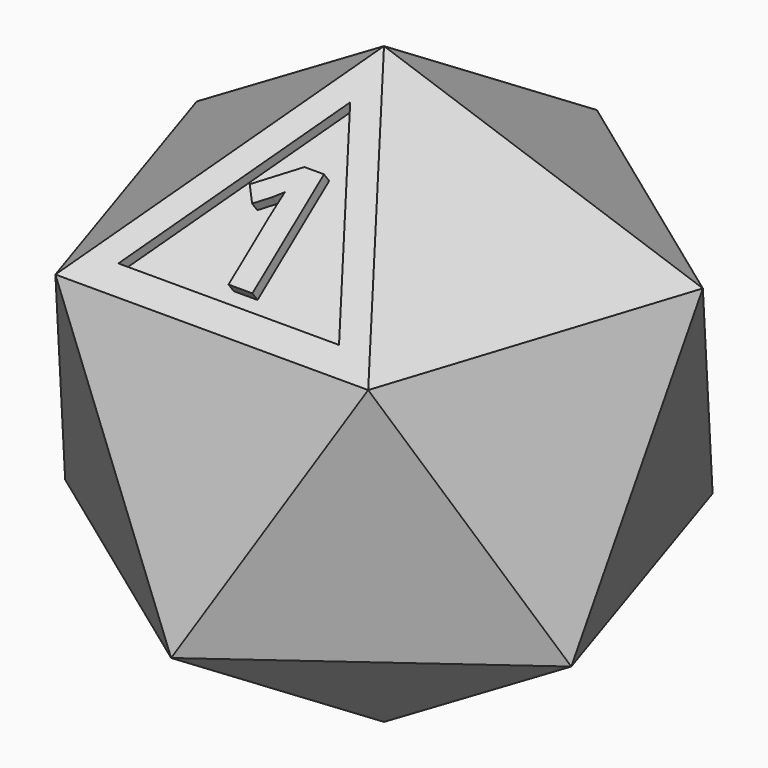
from build123d import *

# Parameters (mm, degrees)
F12_DEPTH      = 37.3243635206
F12_DEPTH_BACK = 37.3243635206
F15_DEPTH      = 37.3243635206
F15_DEPTH_BACK = 37.3243635206
F18_DEPTH      = 37.3243635206
F18_DEPTH_BACK = 37.3243635206
F21_DEPTH      = 37.3243635206
F21_DEPTH_BACK = 37.3243635206
F24_DEPTH      = 37.3243635206
F24_DEPTH_BACK = 37.3243635206
F28_DEPTH      = 99.1671965959
F28_DEPTH_BACK = 99.1671965959
F32_DEPTH      = 89.4601183415
F32_DEPTH_BACK = 89.4601183415
F35_DEPTH      = 89.4601183415
F35_DEPTH_BACK = 88.5596960493
F39_DEPTH      = 99.1671965959
F39_DEPTH_BACK = 96.8098604305
F42_DEPTH      = 68.0823305395
F42_DEPTH_BACK = 70.9961582856
F45_DEPTH      = 92.4043169267
F45_DEPTH_BACK = 99.1671965959
F48_DEPTH      = 81.4313769211
F48_DEPTH_BACK = 89.4601183415
F52_DEPTH      = 88.5596960493
F52_DEPTH_BACK = 82.3317992133
F56_DEPTH      = 92.4043169267
F56_DEPTH_BACK = 96.8098604305
F59_DEPTH      = 68.0823305395
F59_DEPTH_BACK = 68.0823305395
F62_DEPTH      = 37.3243635206
F62_DEPTH_BACK = 37.3243635206
F65_DEPTH      = 68.0823305395
F65_DEPTH_BACK = 68.0823305395
F68_DEPTH      = 81.4313769211
F68_DEPTH_BACK = 81.4313769211
F71_DEPTH      = 92.4043169267
F71_DEPTH_BACK = 92.4043169267
F74_DEPTH      = 92.4043169267
F74_DEPTH_BACK = 92.4043169267
F76_DEPTH      = 2.54
F78_DEPTH      = 2.54


# Not quite as in the source:
# - a feature names something its author has since deleted; it is built from what else it names


with BuildPart() as f9:
    # F7 (on Front) → F9 (revolve)
    with BuildSketch(Plane.XZ):
        with BuildLine():
            Line((0, 0), (0, 31.75))
            Line((0, 31.75), (0, 70.9951582856))
            ThreePointArc((0, 70.9951582856), (-70.9951582856, 0), (0, -70.9951582856))
            Line((0, -70.9951582856), (0, -31.75))
            Line((0, -31.75), (0, 0))
        make_face()
    revolve(axis=Axis((0, 0, -35.4975791428), (0, 0, -1)))

    # F11 (on 3pt) → F12 (cut, two sides)
    with BuildSketch(Plane(origin=(0, 0, 0), x_dir=(-0.5877852523, 0.8090169944, 0), z_dir=(0.8090169944, 0.5877852523, 0))) as f12_sk:
        Polygon((-63.5, -70.9951582856), (0, -70.9951582856), (-51.3725791428, -31.75), (-63.5, -31.75), align=None)
    extrude(amount=F12_DEPTH, mode=Mode.SUBTRACT)
    extrude(f12_sk.sketch, amount=-F12_DEPTH_BACK, mode=Mode.SUBTRACT)

    # F14 (on 3pt) → F15 (cut, two sides)
    with BuildSketch(Plane(origin=(0, 0, 0), x_dir=(-0.5877852523, -0.8090169944, 0), z_dir=(-0.8090169944, 0.5877852523, 0))) as f15_sk:
        Polygon((51.3725791428, -31.75), (0, -70.9951582856), (63.5, -70.9951582856), (63.5, -31.75), align=None)
    extrude(amount=-F15_DEPTH, mode=Mode.SUBTRACT)
    extrude(f15_sk.sketch, amount=F15_DEPTH_BACK, mode=Mode.SUBTRACT)

    # F17 (on 3pt) → F18 (cut, two sides)
    with BuildSketch(Plane(origin=(0, 0, 0), x_dir=(0.9510565163, -0.3090169944, 0), z_dir=(-0.3090169944, -0.9510565163, 0))) as f18_sk:
        Polygon((-63.5, -70.9951582856), (0, -70.9951582856), (-51.3725791428, -31.75), (-63.5, -31.75), align=None)
    extrude(amount=-F18_DEPTH, mode=Mode.SUBTRACT)
    extrude(f18_sk.sketch, amount=F18_DEPTH_BACK, mode=Mode.SUBTRACT)

    # F20 (on 3pt) → F21 (cut, two sides)
    with BuildSketch(Plane.YZ) as f21_sk:
        Polygon((51.3725791428, -31.75), (0, -70.9951582856), (63.5, -70.9951582856), (63.5, -31.75), align=None)
    extrude(amount=-F21_DEPTH, mode=Mode.SUBTRACT)
    extrude(f21_sk.sketch, amount=F21_DEPTH_BACK, mode=Mode.SUBTRACT)

    # F23 (on 3pt) → F24 (cut, two sides)
    with BuildSketch(Plane(origin=(0, 0, 0), x_dir=(-0.9510565163, -0.3090169944, 0), z_dir=(-0.3090169944, 0.9510565163, 0))) as f24_sk:
        Polygon((-63.5, -70.9951582856), (0, -70.9951582856), (-51.3725791428, -31.75), (-63.5, -31.75), align=None)
    extrude(amount=F24_DEPTH, mode=Mode.SUBTRACT)
    extrude(f24_sk.sketch, amount=-F24_DEPTH_BACK, mode=Mode.SUBTRACT)

    # F27 (on 3pt) → F28 (cut, two sides)
    with BuildSketch(Plane(origin=(0, 0, 0), x_dir=(-0.5877852523, 0.8090169944, 0), z_dir=(0.8090169944, 0.5877852523, 0))) as f28_sk:
        Polygon((-70.9951582856, -31.75), (-51.3725791428, -31.75), (-63.5, 31.75), (-70.9951582856, 31.75), align=None)
    extrude(amount=F28_DEPTH, mode=Mode.SUBTRACT)
    extrude(f28_sk.sketch, amount=-F28_DEPTH_BACK, mode=Mode.SUBTRACT)

    # F31 (on 3pt) → F32 (cut, two sides)
    with BuildSketch(Plane(origin=(0, 0, 0), x_dir=(0.9510565163, -0.3090169944, 0), z_dir=(-0.3090169944, -0.9510565163, 0))) as f32_sk:
        Polygon((70.9951582856, 31.75), (51.3725791428, 31.75), (63.5, -31.75), (70.9951582856, -31.75), align=None)
    extrude(amount=-F32_DEPTH, mode=Mode.SUBTRACT)
    extrude(f32_sk.sketch, amount=F32_DEPTH_BACK, mode=Mode.SUBTRACT)

    # F34 (on 3pt) → F35 (cut, two sides)
    with BuildSketch(Plane(origin=(0, 0, 0), x_dir=(0.9510565163, 0.3090169944, 0), z_dir=(0.3090169944, -0.9510565163, 0))) as f35_sk:
        Polygon((63.5, 31.75), (51.3725791428, -31.75), (70.9951582856, -31.75), (70.9951582856, 31.75), align=None)
    extrude(amount=-F35_DEPTH, mode=Mode.SUBTRACT)
    extrude(f35_sk.sketch, amount=F35_DEPTH_BACK, mode=Mode.SUBTRACT)

    # F38 (on 3pt) → F39 (cut, two sides)
    with BuildSketch(Plane(origin=(0, 0, 0), x_dir=(0.5877852523, 0.8090169944, 0), z_dir=(0.8090169944, -0.5877852523, 0))) as f39_sk:
        Polygon((70.9951582856, 31.75), (51.3725791428, 31.75), (63.5, -31.75), (70.9951582856, -31.75), align=None)
    extrude(amount=-F39_DEPTH, mode=Mode.SUBTRACT)
    extrude(f39_sk.sketch, amount=F39_DEPTH_BACK, mode=Mode.SUBTRACT)

    # F41 (on 3pt) → F42 (cut, two sides)
    with BuildSketch(Plane(origin=(0, 0, 0), x_dir=(0, -1, 0), z_dir=(-1, 0, 0))) as f42_sk:
        Polygon((-70.9951582856, -31.75), (-51.3725791428, -31.75), (-63.5, 31.75), (-70.9951582856, 31.75), align=None)
    extrude(amount=-F42_DEPTH, mode=Mode.SUBTRACT)
    extrude(f42_sk.sketch, amount=F42_DEPTH_BACK, mode=Mode.SUBTRACT)

    # F44 (on 3pt) → F45 (cut, two sides)
    with BuildSketch(Plane(origin=(0, 0, 0), x_dir=(0.5877852523, -0.8090169944, 0), z_dir=(-0.8090169944, -0.5877852523, 0))) as f45_sk:
        Polygon((-63.5, -31.75), (-51.3725791428, 31.75), (-70.9951582856, 31.75), (-70.9951582856, -31.75), align=None)
    extrude(amount=-F45_DEPTH, mode=Mode.SUBTRACT)
    extrude(f45_sk.sketch, amount=F45_DEPTH_BACK, mode=Mode.SUBTRACT)

    # F47 (on 3pt) → F48 (cut, two sides)
    with BuildSketch(Plane(origin=(0, 0, 0), x_dir=(0.9510565163, -0.3090169944, 0), z_dir=(-0.3090169944, -0.9510565163, 0))) as f48_sk:
        Polygon((-70.9951582856, -31.75), (-51.3725791428, -31.75), (-63.5, 31.75), (-70.9951582856, 31.75), align=None)
    extrude(amount=-F48_DEPTH, mode=Mode.SUBTRACT)
    extrude(f48_sk.sketch, amount=F48_DEPTH_BACK, mode=Mode.SUBTRACT)

    # F51 (on 3pt) → F52 (cut, two sides)
    with BuildSketch(Plane(origin=(0, 0, 0), x_dir=(-0.9510565163, -0.3090169944, 0), z_dir=(-0.3090169944, 0.9510565163, 0))) as f52_sk:
        Polygon((70.9951582856, 31.75), (51.3725791428, 31.75), (63.5, -31.75), (70.9951582856, -31.75), align=None)
    extrude(amount=-F52_DEPTH, mode=Mode.SUBTRACT)
    extrude(f52_sk.sketch, amount=F52_DEPTH_BACK, mode=Mode.SUBTRACT)

    # F55 (on 3pt) → F56 (cut, two sides)
    with BuildSketch(Plane(origin=(0, 0, 0), x_dir=(0.5877852523, 0.8090169944, 0), z_dir=(0.8090169944, -0.5877852523, 0))) as f56_sk:
        Polygon((-70.9951582856, -31.75), (-51.3725791428, -31.75), (-63.5, 31.75), (-70.9951582856, 31.75), align=None)
    extrude(amount=-F56_DEPTH, mode=Mode.SUBTRACT)
    extrude(f56_sk.sketch, amount=F56_DEPTH_BACK, mode=Mode.SUBTRACT)

    # F58 (on 3pt) → F59 (cut, two sides)
    with BuildSketch(Plane(origin=(0, 0, 0), x_dir=(0, -1, 0), z_dir=(-1, 0, 0))) as f59_sk:
        Polygon((70.9951582856, 31.75), (51.3725791428, 31.75), (63.5, -31.75), (70.9951582856, -31.75), align=None)
    extrude(amount=-F59_DEPTH, mode=Mode.SUBTRACT)
    extrude(f59_sk.sketch, amount=F59_DEPTH_BACK, mode=Mode.SUBTRACT)

    # F61 (on 3pt) → F62 (cut, two sides)
    with BuildSketch(Plane(origin=(0, 0, 0), x_dir=(0.9510565163, -0.3090169944, 0), z_dir=(-0.3090169944, -0.9510565163, 0))) as f62_sk:
        Polygon((63.5, 70.9951582856), (0, 70.9951582856), (51.3725791428, 31.75), (63.5, 31.75), align=None)
    extrude(amount=F62_DEPTH, mode=Mode.SUBTRACT)
    extrude(f62_sk.sketch, amount=-F62_DEPTH_BACK, mode=Mode.SUBTRACT)

    # F64 (on 3pt) → F65 (cut, two sides)
    with BuildSketch(Plane.YZ) as f65_sk:
        Polygon((-51.3725791428, 31.75), (0, 70.9951582856), (-63.5, 70.9951582856), (-63.5, 31.75), align=None)
    extrude(amount=-F65_DEPTH, mode=Mode.SUBTRACT)
    extrude(f65_sk.sketch, amount=F65_DEPTH_BACK, mode=Mode.SUBTRACT)

    # F67 (on 3pt) → F68 (cut, two sides)
    with BuildSketch(Plane(origin=(0, 0, 0), x_dir=(0.9510565163, 0.3090169944, 0), z_dir=(0.3090169944, -0.9510565163, 0))) as f68_sk:
        Polygon((-51.3725791428, 31.75), (0, 70.9951582856), (-63.5, 70.9951582856), (-63.5, 31.75), align=None)
    extrude(amount=-F68_DEPTH, mode=Mode.SUBTRACT)
    extrude(f68_sk.sketch, amount=F68_DEPTH_BACK, mode=Mode.SUBTRACT)

    # F70 (on 3pt) → F71 (cut, two sides)
    with BuildSketch(Plane(origin=(0, 0, 0), x_dir=(-0.5877852523, 0.8090169944, 0), z_dir=(0.8090169944, 0.5877852523, 0))) as f71_sk:
        Polygon((63.5, 70.9951582856), (0, 70.9951582856), (51.3725791428, 31.75), (63.5, 31.75), align=None)
    extrude(amount=-F71_DEPTH, mode=Mode.SUBTRACT)
    extrude(f71_sk.sketch, amount=F71_DEPTH_BACK, mode=Mode.SUBTRACT)

    # F73 (on 3pt) → F74 (cut, two sides)
    with BuildSketch(Plane(origin=(0, 0, 0), x_dir=(0.5877852523, 0.8090169944, 0), z_dir=(0.8090169944, -0.5877852523, 0))) as f74_sk:
        Polygon((63.5, 70.9951582856), (0, 70.9951582856), (51.3725791428, 31.75), (63.5, 31.75), align=None)
    extrude(amount=-F74_DEPTH, mode=Mode.SUBTRACT)
    extrude(f74_sk.sketch, amount=F74_DEPTH_BACK, mode=Mode.SUBTRACT)

    # F75 (on face) → F76 (cut)
    with BuildSketch(Plane(origin=(0, -34.2483860952, 44.8317194285), x_dir=(1, 0, 0), z_dir=(0, -0.6070619982, 0.7946544723))):
        Polygon((26.3258408925, -15.1992313259), (0, 30.3984626519), (-26.3258408925, -15.1992313259), align=None)
        with BuildLine():
            Line((3.3501555036, 15.3069211224), (3.3501555036, -11.5860768557))
            Line((3.3501555036, -11.5860768557), (-2.335691738, -11.5860768557))
            Line((-2.335691738, -11.5860768557), (-2.335691738, 3.9764284308))
            Line((-2.335691738, 3.9764284308), (-2.2768320357, 6.5309395104))
            Line((-2.2768320357, 6.5309395104), (-2.1885424823, 9.3267753694))
            add(Edge.make_bspline(
                [(-2.1885424823, 9.3267753694), (-3.6011753374, 7.9141425143), (-4.1544565389, 7.4726947471)],
                knots=[0, 0, 0, 1, 1, 1], degree=2))
            Line((-4.1544565389, 7.4726947471), (-7.2445909094, 4.9888153103))
            Line((-7.2445909094, 4.9888153103), (-9.9874530363, 8.4085640136))
            Line((-9.9874530363, 8.4085640136), (-1.3233048586, 15.3069211224))
            Line((-1.3233048586, 15.3069211224), (3.3501555036, 15.3069211224))
        make_face(mode=Mode.SUBTRACT)
    extrude(amount=-F76_DEPTH, mode=Mode.SUBTRACT)

    # F77 (on face) → F78 (cut)
    with BuildSketch(Plane(origin=(0, 34.2483860952, -44.8317194285), x_dir=(1, 0, 0), z_dir=(0, 0.6070619982, -0.7946544723))):
        with BuildLine():
            Line((26.3258408925, -15.1992313259), (0, 30.3984626519))
            Line((0, 30.3984626519), (-11.6958512292, 10.1406540851))
            add(Edge.make_bspline(
                [(-11.6958512292, 10.1406540851), (-10.9085633152, 10.5210577591), (-10.0027118644, 10.7419129699)],
                knots=[0.151662927, 0.151662927, 0.151662927, 1, 1, 1], degree=2))
            add(Edge.make_bspline(
                [(-10.0027118644, 10.7419129699), (-8.9349152542, 11.002251953), (-7.6128813559, 11.002251953)],
                knots=[0, 0, 0, 1, 1, 1], degree=2))
            add(Edge.make_bspline(
                [(-7.6128813559, 11.002251953), (-5.8718644068, 11.002251953), (-4.5376271186, 10.3676756818)],
                knots=[0, 0, 0, 1, 1, 1], degree=2))
            add(Edge.make_bspline(
                [(-4.5376271186, 10.3676756818), (-3.2033898305, 9.7330994106), (-2.4650847458, 8.5880146649)],
                knots=[0, 0, 0, 1, 1, 1], degree=2))
            add(Edge.make_bspline(
                [(-2.4650847458, 8.5880146649), (-1.726779661, 7.4429299191), (-1.726779661, 5.9703875462)],
                knots=[0, 0, 0, 1, 1, 1], degree=2))
            add(Edge.make_bspline(
                [(-1.726779661, 5.9703875462), (-1.726779661, 4.6849638174), (-2.1783050847, 3.5602180547)],
                knots=[0, 0, 0, 1, 1, 1], degree=2))
            add(Edge.make_bspline(
                [(-2.1783050847, 3.5602180547), (-2.6298305085, 2.435472292), (-3.5776271186, 1.2537773767)],
                knots=[0, 0, 0, 1, 1, 1], degree=2))
            add(Edge.make_bspline(
                [(-3.5776271186, 1.2537773767), (-4.5254237288, 0.0720824615), (-6.913220339, -2.1163921148)],
                knots=[0, 0, 0, 1, 1, 1], degree=2))
            Line((-6.913220339, -2.1163921148), (-9.3050847458, -4.3658836402))
            Line((-9.3050847458, -4.3658836402), (-9.3050847458, -4.5407988945))
            Line((-9.3050847458, -4.5407988945), (-1.2061016949, -4.5407988945))
            Line((-1.2061016949, -4.5407988945), (-1.2061016949, -7.8479175385))
            Line((-1.2061016949, -7.8479175385), (-14.1986440678, -7.8479175385))
            Line((-14.1986440678, -7.8479175385), (-14.1986440678, -5.1143582165))
            Line((-14.1986440678, -5.1143582165), (-9.5328813559, -0.3997819453))
            add(Edge.make_bspline(
                [(-9.5328813559, -0.3997819453), (-7.4583050847, 1.7236078852), (-6.8237288136, 2.5432689022)],
                knots=[0, 0, 0, 1, 1, 1], degree=2))
            add(Edge.make_bspline(
                [(-6.8237288136, 2.5432689022), (-6.1891525424, 3.3629299191), (-5.9084745763, 4.0625909361)],
                knots=[0, 0, 0, 1, 1, 1], degree=2))
            add(Edge.make_bspline(
                [(-5.9084745763, 4.0625909361), (-5.6277966102, 4.762251953), (-5.6277966102, 5.5107265293)],
                knots=[0, 0, 0, 1, 1, 1], degree=2))
            add(Edge.make_bspline(
                [(-5.6277966102, 5.5107265293), (-5.6277966102, 6.6293705971), (-6.2461016949, 7.1764892411)],
                knots=[0, 0, 0, 1, 1, 1], degree=2))
            add(Edge.make_bspline(
                [(-6.2461016949, 7.1764892411), (-6.8644067797, 7.7236078852), (-7.893559322, 7.7236078852)],
                knots=[0, 0, 0, 1, 1, 1], degree=2))
            add(Edge.make_bspline(
                [(-7.893559322, 7.7236078852), (-8.9715254237, 7.7236078852), (-9.9884745763, 7.2273366988)],
                knots=[0, 0, 0, 1, 1, 1], degree=2))
            add(Edge.make_bspline(
                [(-9.9884745763, 7.2273366988), (-11.0054237288, 6.7310655123), (-12.1118644068, 5.815811275)],
                knots=[0, 0, 0, 1, 1, 1], degree=2))
            Line((-12.1118644068, 5.815811275), (-13.3475580235, 7.2798139981))
            Line((-13.3475580235, 7.2798139981), (-26.3258408925, -15.1992313259))
            Line((-26.3258408925, -15.1992313259), (26.3258408925, -15.1992313259))
        make_face()
        with BuildLine():
            add(Edge.make_bspline(
                [(11.906440678, 8.5900485632), (13.5518644068, 6.1493705971), (13.5518644068, 1.4429299191)],
                knots=[0, 0, 0, 1, 1, 1], degree=2))
            add(Edge.make_bspline(
                [(13.5518644068, 1.4429299191), (13.5518644068, -3.4221548267), (11.9572881356, -5.7631717758)],
                knots=[0, 0, 0, 1, 1, 1], degree=2))
            add(Edge.make_bspline(
                [(11.9572881356, -5.7631717758), (10.3627118644, -8.104188725), (7.0433898305, -8.104188725)],
                knots=[0, 0, 0, 1, 1, 1], degree=2))
            add(Edge.make_bspline(
                [(7.0433898305, -8.104188725), (3.8257627119, -8.104188725), (2.1925423729, -5.6879175385)],
                knots=[0, 0, 0, 1, 1, 1], degree=2))
            add(Edge.make_bspline(
                [(2.1925423729, -5.6879175385), (0.5593220339, -3.2716463521), (0.5593220339, 1.4429299191)],
                knots=[0, 0, 0, 1, 1, 1], degree=2))
            add(Edge.make_bspline(
                [(0.5593220339, 1.4429299191), (0.5593220339, 6.3649638174), (2.1498305085, 8.6978451733)],
                knots=[0, 0, 0, 1, 1, 1], degree=2))
            add(Edge.make_bspline(
                [(2.1498305085, 8.6978451733), (3.7403389831, 11.0307265293), (7.0433898305, 11.0307265293)],
                knots=[0, 0, 0, 1, 1, 1], degree=2))
            add(Edge.make_bspline(
                [(7.0433898305, 11.0307265293), (10.2610169492, 11.0307265293), (11.906440678, 8.5900485632)],
                knots=[0, 0, 0, 1, 1, 1], degree=2))
        make_face(mode=Mode.SUBTRACT)
        with BuildLine():
            add(Edge.make_bspline(
                [(5.0603389831, 6.3568282242), (4.4644067797, 4.8639468683), (4.4644067797, 1.4429299191)],
                knots=[0, 0, 0, 1, 1, 1], degree=2))
            add(Edge.make_bspline(
                [(4.4644067797, 1.4429299191), (4.4644067797, -1.9740192334), (5.0542372881, -3.4546971995)],
                knots=[0, 0, 0, 1, 1, 1], degree=2))
            add(Edge.make_bspline(
                [(5.0542372881, -3.4546971995), (5.6440677966, -4.9353751656), (7.0433898305, -4.9353751656)],
                knots=[0, 0, 0, 1, 1, 1], degree=2))
            add(Edge.make_bspline(
                [(7.0433898305, -4.9353751656), (8.4183050847, -4.9353751656), (9.0284745763, -3.4363921148)],
                knots=[0, 0, 0, 1, 1, 1], degree=2))
            add(Edge.make_bspline(
                [(9.0284745763, -3.4363921148), (9.6386440678, -1.9374090639), (9.6386440678, 1.4429299191)],
                knots=[0, 0, 0, 1, 1, 1], degree=2))
            add(Edge.make_bspline(
                [(9.6386440678, 1.4429299191), (9.6386440678, 4.8639468683), (9.0203389831, 6.3568282242)],
                knots=[0, 0, 0, 1, 1, 1], degree=2))
            add(Edge.make_bspline(
                [(9.0203389831, 6.3568282242), (8.4020338983, 7.8497095801), (7.0433898305, 7.8497095801)],
                knots=[0, 0, 0, 1, 1, 1], degree=2))
            add(Edge.make_bspline(
                [(7.0433898305, 7.8497095801), (5.6562711864, 7.8497095801), (5.0603389831, 6.3568282242)],
                knots=[0, 0, 0, 1, 1, 1], degree=2))
        make_face()
    extrude(amount=-F78_DEPTH, mode=Mode.SUBTRACT)


solid = f9.part
